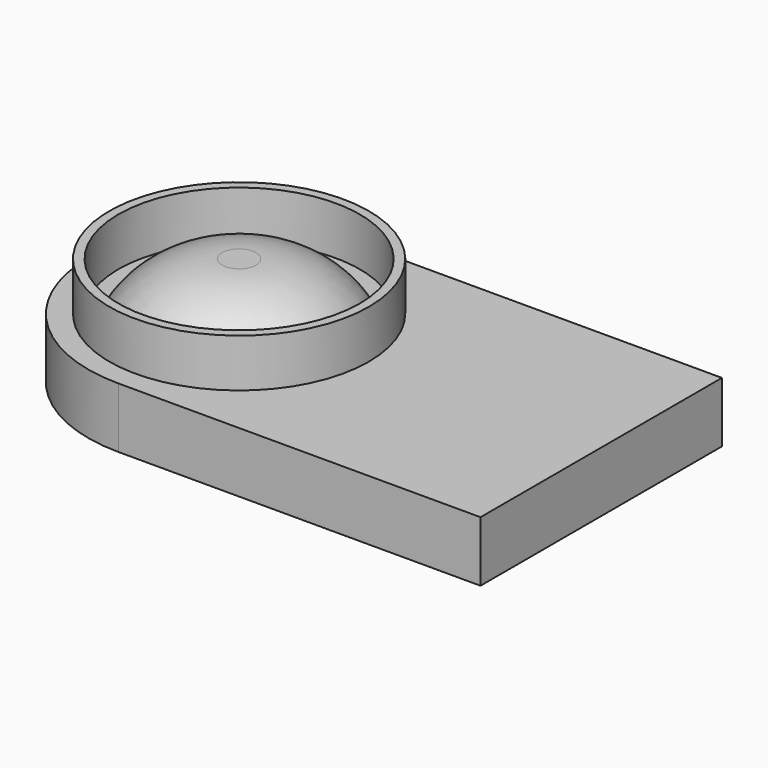
from build123d import *

# Parameters (mm, degrees)
F0_R     = 21.5
F0_R_2   = 20
F0_R_3   = 17.5
F1_DEPTH = 10
F2_DEPTH = 8
F3_DEPTH = 8


# Not quite as in the source:
# - a fillet or chamfer that OpenCascade refuses, or shapes differently, is made with other operations: its cross-section is extruded or revolved along the edge and cut away or added


with BuildPart() as f1:
    # F0 (on Top) → F1 (new body)
    with BuildSketch(Plane.XY):
        with BuildLine():
            Line((60, 25), (0, 25))
            ThreePointArc((0, 25), (-25, 0), (0, -25))
            Line((0, -25), (60, -25))
            Line((60, -25), (60, 25))
        make_face()
        Circle(F0_R, mode=Mode.SUBTRACT)
        Circle(F0_R)
        Circle(F0_R_2, mode=Mode.SUBTRACT)
        Circle(F0_R_2)
        Circle(F0_R_3, mode=Mode.SUBTRACT)
        Circle(F0_R_3)
    extrude(amount=-F1_DEPTH)


with BuildPart() as f2:
    # F0 (on Top) → F2 (new body)
    with BuildSketch(Plane.XY):
        Circle(F0_R)
        Circle(F0_R_2, mode=Mode.SUBTRACT)
    extrude(amount=F2_DEPTH)


with BuildPart() as f3:
    # F0 (on Top) → F3 (new body)
    with BuildSketch(Plane.XY):
        Circle(F0_R_3)
    extrude(amount=F3_DEPTH)

    # F4: fillet of radius 17.5 on 1 edges, made by hand

    # F4_s1 → F4_t2 (revolve, cut)
    with BuildSketch(Plane.XZ):
        with BuildLine():
            ThreePointArc((17.5, 0), (11.1696618086, 5.8704261489), (2.8030615433, 8))
            Line((2.8030615433, 8), (17.5, 8))
            Line((17.5, 8), (17.5, 0))
        make_face()
    revolve(axis=Axis((0, 0, 8), (0, 0, 1)), mode=Mode.SUBTRACT)


solid = Compound([f1.part, f2.part, f3.part])
